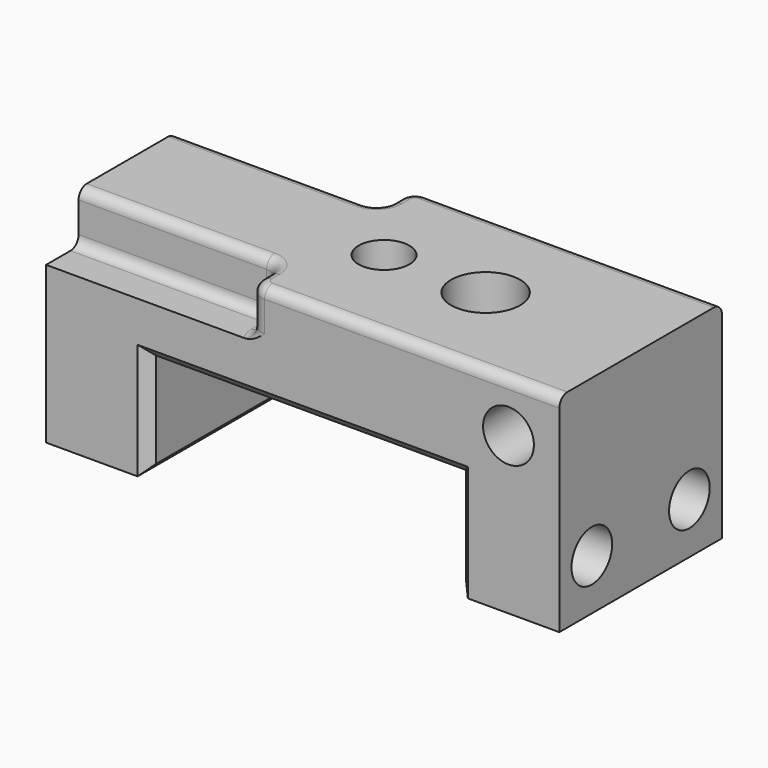
from build123d import *

# Parameters (mm, degrees)
F1_DEPTH       = 10
F5_D           = 5
F5_DEPTH       = 8
F5_TIP         = 1.5021515476
F5_ON_F4_D     = 5
F5_ON_F4_DEPTH = 8
F5_ON_F4_TIP   = 1.5021515476
F6_D           = 6.8
F6_DEPTH       = 19
F6_TIP         = 2.0429261047
F8_D           = 4.2
F8_DEPTH       = 10
F8_TIP         = 1.2618073
F10_D          = 5
F10_DEPTH      = 20
F10_TIP        = 1.5021515476
F13_D          = 6.8
F13_DEPTH      = 7
F13_TIP        = 2.0429261047
F14_D          = 5
F14_DEPTH      = 8
F14_TIP        = 1.5021515476
F16_DEPTH      = 5
F17_SIZE       = 1
F18_F1_R       = 1
F18_F2_R       = 1
F18_F3_R       = 1
F18_F4_R       = 1


# Not quite as in the source:
# - a feature names something its author has since deleted; it is built from what else it names


with BuildPart() as f1:
    # F0 (on Front) → F1 (new body, symmetric)
    with BuildSketch(Plane.XZ):
        Polygon((-25.25, 0), (-25.25, -20.4), (-15.25, -20.4), (-15.25, -10), (15.25, -10), (15.25, -20.4), (25.25, -20.4), (25.25, 0), align=None)
    extrude(amount=F1_DEPTH, both=True)

    # F5
    with Locations(Plane(origin=(-25.25, 0, 0), x_dir=(0, -1, 0), z_dir=(-1, 0, 0))):
        with Locations((6, -15.4), (-6, -15.4)):
            Hole(F5_D / 2, depth=F5_DEPTH)
            with Locations((0, 0, -(F5_DEPTH + F5_TIP / 2))):  # 118° drill point
                Cone(0, F5_D / 2, F5_TIP, mode=Mode.SUBTRACT)

    # F5 on F4
    with Locations(Plane.YZ.offset(25.25)):
        with Locations((-6, -15.4), (6, -15.4)):
            Hole(F5_ON_F4_D / 2, depth=F5_ON_F4_DEPTH)
            with Locations((0, 0, -(F5_ON_F4_DEPTH + F5_ON_F4_TIP / 2))):  # 118° drill point
                Cone(0, F5_ON_F4_D / 2, F5_ON_F4_TIP, mode=Mode.SUBTRACT)

    # F6
    with Locations(Plane(origin=(-25.25, 0, 0), x_dir=(0, -1, 0), z_dir=(-1, 0, 0))):
        with Locations((0, -5)):
            Hole(F6_D / 2, depth=F6_DEPTH)
            with Locations((0, 0, -(F6_DEPTH + F6_TIP / 2))):  # 118° drill point
                Cone(0, F6_D / 2, F6_TIP, mode=Mode.SUBTRACT)

    # F8
    with Locations(Plane(origin=(0, 0, -20.4), x_dir=(1, 0, 0), z_dir=(0, 0, -1))):
        with Locations((-20.25, 0), (20.25, 0)):
            Hole(F8_D / 2, depth=F8_DEPTH)
            with Locations((0, 0, -(F8_DEPTH + F8_TIP / 2))):  # 118° drill point
                Cone(0, F8_D / 2, F8_TIP, mode=Mode.SUBTRACT)

    # F10
    with Locations(Plane.XZ.offset(10)):
        with Locations((20.25, -5)):
            Hole(F10_D / 2, depth=F10_DEPTH)
            with Locations((0, 0, -(F10_DEPTH + F10_TIP / 2))):  # 118° drill point
                Cone(0, F10_D / 2, F10_TIP, mode=Mode.SUBTRACT)

    # F13
    with Locations(Plane.XY):
        with Locations((10, 0)):
            Hole(F13_D / 2, depth=F13_DEPTH)
            with Locations((0, 0, -(F13_DEPTH + F13_TIP / 2))):  # 118° drill point
                Cone(0, F13_D / 2, F13_TIP, mode=Mode.SUBTRACT)

    # F14
    with Locations(Plane.XY):
        with Locations((0, 0)):
            Hole(F14_D / 2, depth=F14_DEPTH)
            with Locations((0, 0, -(F14_DEPTH + F14_TIP / 2))):  # 118° drill point
                Cone(0, F14_D / 2, F14_TIP, mode=Mode.SUBTRACT)

    # F15 (on face) → F16 (cut)
    with BuildSketch(Plane.XY):
        with BuildLine():
            Line((-6.75, -6), (-25.25, -6))
            Line((-25.25, -6), (-25.25, -10))
            Line((-25.25, -10), (-3.75, -10))
            ThreePointArc((-3.75, -10), (-4.8106601718, -9.5606601718), (-5.25, -8.5))
            Line((-5.25, -8.5), (-5.25, -7.5))
            ThreePointArc((-5.25, -7.5), (-5.6893398282, -6.4393398282), (-6.75, -6))
        make_face()
        with BuildLine():
            Line((-25.25, 10), (-25.25, 6))
            Line((-25.25, 6), (-6.75, 6))
            ThreePointArc((-6.75, 6), (-5.6893398282, 6.4393398282), (-5.25, 7.5))
            Line((-5.25, 7.5), (-5.25, 8.5))
            ThreePointArc((-5.25, 8.5), (-4.8106601718, 9.5606601718), (-3.75, 10))
            Line((-3.75, 10), (-25.25, 10))
        make_face()
    extrude(amount=-F16_DEPTH, mode=Mode.SUBTRACT)

    # F17
    f17_edges = [f1.edges().sort_by_distance(p)[0] for p in [
        (15.25, 0, -20.4),
        (-15.25, 0, -20.4),
        (-15.25, -10, -15.2),
        (0, -10, -10),
        (15.25, -10, -15.2),
        (0, 10, -10),
        (-15.25, 10, -15.2),
        (15.25, 10, -15.2),
    ]]
    chamfer(f17_edges, length=F17_SIZE)

    # F18: fillet of radius 1 on 16 edges, made by hand

    # F18_f1
    f18_f1_edges = [f1.edges().sort_by_distance(p)[0] for p in [
        (10.75, -10, 0),
        (-4.8106601718, -9.5606601718, 0),
        (-5.25, -8, 0),
        (-5.6893398282, -6.4393398282, 0),
        (-16, -6, 0),
    ]]
    fillet(f18_f1_edges, radius=F18_F1_R)

    # F18_f2
    f18_f2_edges = [f1.edges().sort_by_distance(p)[0] for p in [
        (-16, 6, 0),
        (-5.6893398282, 6.4393398282, 0),
        (-5.25, 8, 0),
        (-4.8106601718, 9.5606601718, 0),
        (10.75, 10, 0),
    ]]
    fillet(f18_f2_edges, radius=F18_F2_R)

    # F18_f3
    f18_f3_edges = [f1.edges().sort_by_distance(p)[0] for p in [
        (-4.8106601718, -9.5606601718, -5),
        (-16, -6, -5),
        (-5.25, -8, -5),
        (-5.6893398282, -6.4393398282, -5),
    ]]
    fillet(f18_f3_edges, radius=F18_F3_R)

    # F18_f4
    f18_f4_edges = [f1.edges().sort_by_distance(p)[0] for p in [
        (-16, 6, -5),
        (-5.6893398282, 6.4393398282, -5),
        (-5.25, 8, -5),
        (-4.8106601718, 9.5606601718, -5),
    ]]
    fillet(f18_f4_edges, radius=F18_F4_R)


solid = f1.part
